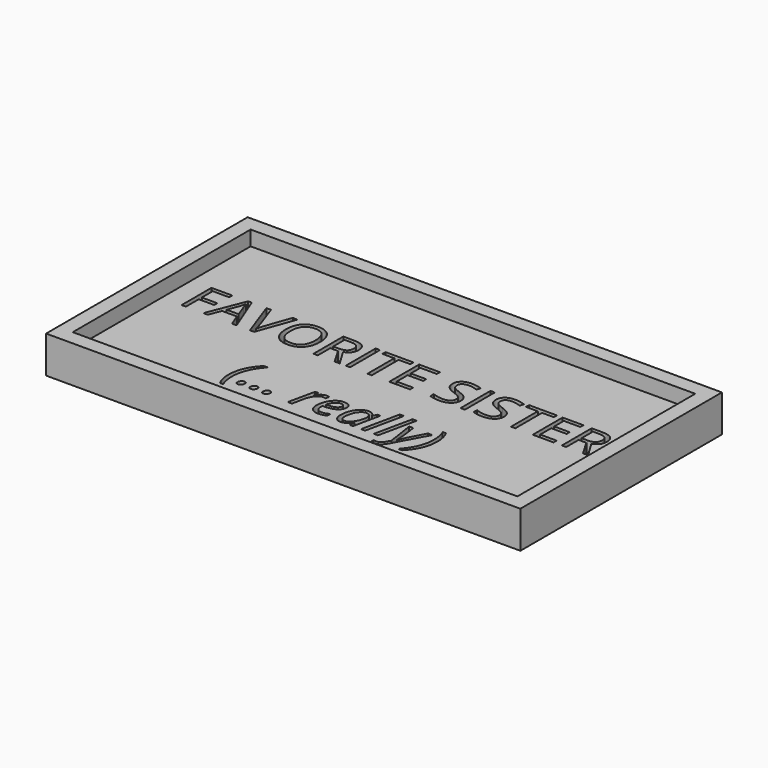
from build123d import *

# Parameters (mm, degrees)
F0_TEXT_SIZE   = 22.3907439838
F0_TEXT_SIZE_2 = 21.5913893448
F1_DEPTH       = 25.4
F2_W           = 203.2
F2_H           = 107.95
F3_DEPTH       = 4.7625
F4_W           = 203.2
F4_H           = 107.95
F5_DEPTH       = 4.7625
F7_W           = 203.2
F7_H           = 107.95
F7_W_2         = 190.5
F7_H_2         = 95.25
F8_DEPTH       = 6.35


# Not quite as in the source:
# - Text() gives the source's letters only with a copy of the font that has no kerning and outlines rounded to 1/6400 em; it was checked with that copy


with BuildPart() as f1:
    # F0 (on Top) → F1 (new body)
    with BuildSketch(Plane.XY):
        with Locations((-88.9, 0)):
            Text('FAVORITE SISTER', F0_TEXT_SIZE, font='Open Sans', text_align=(TextAlign.LEFT, TextAlign.BOTTOM))
        with Locations((-43.8326895237, -32.7063202858)):
            Text('(... really)', F0_TEXT_SIZE_2, font='Open Sans', font_style=FontStyle.ITALIC, text_align=(TextAlign.LEFT, TextAlign.BOTTOM))
    extrude(amount=F1_DEPTH)


with BuildPart() as f3:
    # F2 (on Top) → F3 (new body)
    with BuildSketch(Plane.XY):
        Rectangle(F2_W, F2_H)
    extrude(amount=-F3_DEPTH)

    # F4 (on Top) → F5 (join)
    with BuildSketch(Plane.XY):
        Rectangle(F4_W, F4_H)
    extrude(amount=F5_DEPTH)

    # F6: cut F1
    add(f1.part, mode=Mode.SUBTRACT)

    # F7 (on face) → F8 (join)
    with BuildSketch(Plane.XY.offset(4.7625)):
        Rectangle(F7_W, F7_H)
        Rectangle(F7_W_2, F7_H_2, mode=Mode.SUBTRACT)
    extrude(amount=F8_DEPTH)


solid = f3.part
